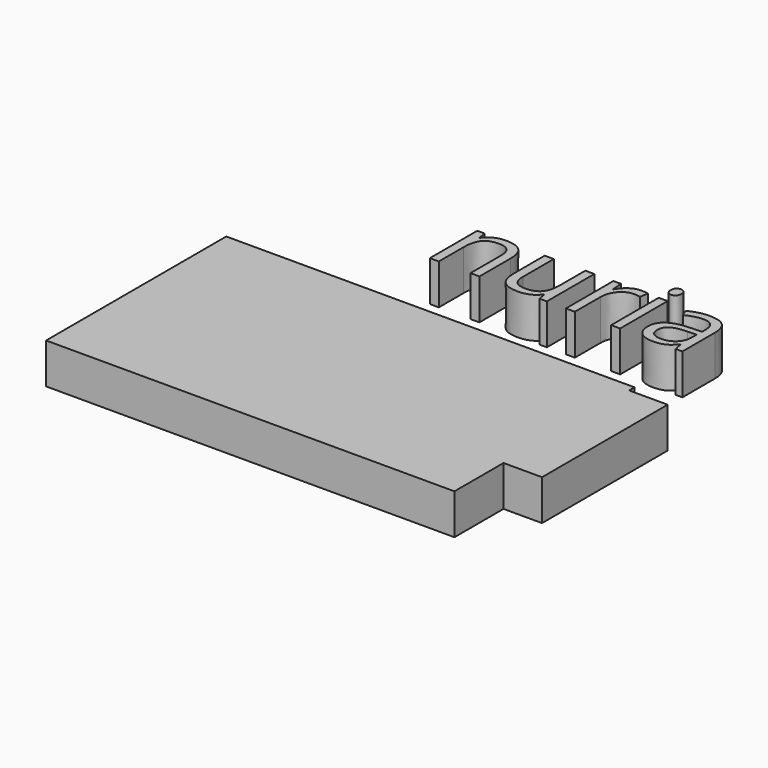
from build123d import *

# Parameters (mm, degrees)
F0_W         = 62.9002302885
F0_H         = 38.8326756656
F0_W_2       = 9.5190964639
F0_TEXT_SIZE = 27.4135834641
F1_DEPTH     = 10


# Not quite as in the source:
# - Text() gives the source's letters only with a copy of the font that has no kerning and outlines rounded to 1/6400 em; it was checked with that copy


with BuildPart() as f1:
    # F0 (on Top) → F1 (new body)
    with BuildSketch(Plane.XY):
        Polygon((-38.2569506764, -20.0607143342), (-38.2569506764, 18.7719613314), (24.6432796121, 18.7719613314), (24.6432796121, 20.4504970461), (-76.3222947717, 20.4504970461), (-76.3222947717, -35.2338403463), (24.6432796121, -35.2338403463), (24.6432796121, -20.0607143342), align=None)
        with Locations((-6.8068355322, -0.6443765014)):
            Rectangle(F0_W, F0_H)
        with Locations((29.402827844, -0.6443765014)):
            Rectangle(F0_W_2, F0_H)
        with Locations((-42.3270612955, 37.9271507263)):
            Text('nuria', F0_TEXT_SIZE, font='Open Sans', text_align=(TextAlign.LEFT, TextAlign.BOTTOM))
    extrude(amount=F1_DEPTH)


solid = f1.part
